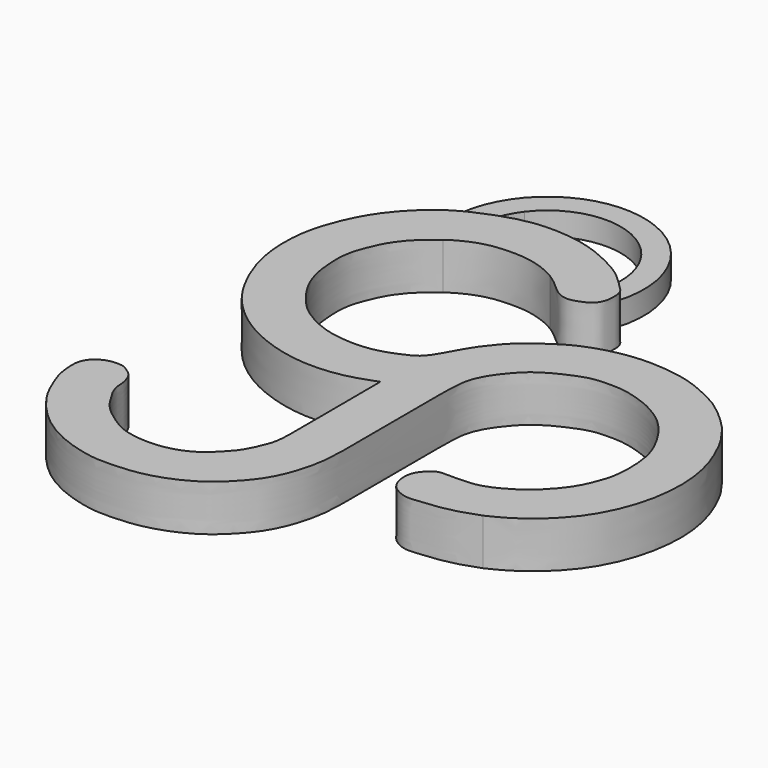
from build123d import *

# Parameters (mm, degrees)
F1_DEPTH = 6
F2_DEPTH = 3


with BuildPart() as f1:
    # F0 (on Top) → F1 (new body)
    with BuildSketch(Plane.XY):
        with BuildLine():
            add(Edge.make_bspline(
                [(-61.713565141, -18.9343132079), (-63.0146348838, -19.4095390469), (-65.733189771, -20.4025123556), (-70.8280130497, -20.6815591765), (-75.7018481976, -19.5041294338), (-80.0931153376, -17.3641610679), (-84.0038443733, -13.8752753533), (-86.4313989815, -9.8518831116), (-88.2796036438, -5.0190108695), (-88.4963736266, 0.0085689786), (-87.8617186152, 3.6375292768), (-86.1935172065, 7.9287613179), (-83.9416658783, 11.1542399806), (-82.1275636618, 12.9283614758), (-81.3241270743, 13.5947379823)],
                knots=[0, 0, 0, 0, 0.0181122524, 0.0378370444, 0.0574807634, 0.0768858202, 0.0968162077, 0.1158466157, 0.1358456208, 0.1553780521, 0.1722749914, 0.190949199, 0.2090855796, 0.2233461087, 0.2233461087, 0.2233461087, 0.2233461087], degree=3))
            add(Edge.make_bspline(
                [(-35.296164453, -35.3126786649), (-35.8181301783, -35.5024037361), (-36.8134666802, -35.8641904962), (-38.0708117456, -36.270480159), (-40.138121174, -36.7077930279), (-42.3688721513, -36.8892351142), (-44.2325900627, -37.1059998289), (-45.7225874453, -36.2585038344), (-46.2929253284, -35.686129434), (-46.7363136163, -34.8014748443), (-46.8692619716, -33.8262575164), (-46.8065307463, -32.7032975926), (-46.2297636494, -31.7451552895), (-45.5431628055, -31.0933682437), (-44.8464319505, -30.5974831217), (-43.7455158564, -30.5822460272), (-42.5044985041, -30.6260654275), (-40.8703078904, -30.5481728825), (-39.8792195184, -30.4326386682), (-38.1797456225, -29.8531864623), (-36.9342661804, -29.1089567426), (-35.3238356448, -28.1904757097), (-33.170383713, -26.07435277), (-31.8582431136, -24.2273615637), (-31.1469842445, -22.6450405096), (-30.3725491148, -20.5779895244), (-30.2104838527, -18.4841397494), (-30.2501485523, -16.3106662094), (-30.6343803225, -13.9306564773), (-31.7748028839, -11.5465745257), (-33.186348835, -9.4322593089), (-34.8104844807, -7.735799033), (-37.1662119159, -6.2493083282), (-39.2182087251, -5.5030771293), (-41.166575858, -4.9558334521), (-42.9870195119, -4.859445306), (-45.4834836068, -4.897725137), (-47.7441223228, -5.8310077864), (-49.5208260418, -6.6596538791), (-51.4234507273, -7.8666605714), (-53.073082843, -9.7195908219), (-54.248737469, -11.3737650388), (-54.997105148, -13.1154447546), (-55.2687748261, -15.0229815759), (-55.2632841388, -20.2243601486), (-55.2042759513, -27.8226519462), (-55.2098481, -33.936082992), (-55.4095257107, -36.7774227554), (-56.4540380047, -40.5834941392), (-57.9776164972, -43.2587210437), (-59.7304487982, -45.2135126916), (-61.4142605805, -46.8277136166), (-63.9910912681, -48.4006874678), (-66.4861437494, -49.3100674413), (-68.5320453717, -49.8112197331), (-70.8281422598, -50.0305338543), (-73.6749221598, -50.1055434421), (-76.0600796044, -49.5953323554), (-78.2545980933, -48.9285309184), (-80.3394186289, -47.94916046), (-82.3766699977, -46.6394319711), (-84.5941350037, -44.5319080526), (-86.5559834995, -41.9402439855), (-87.7388820002, -38.9490920475), (-88.223461995, -37.5450863847), (-88.4518870314, -35.3054185599), (-88.1689144899, -33.996902953), (-87.2535647901, -32.9598891209), (-86.064578952, -32.4525417401), (-85.2012031694, -32.3805571825), (-84.1562979368, -32.3779337124), (-83.4415258264, -32.8900691989), (-82.5667565857, -33.4633434329), (-82.1276496152, -34.4287627257), (-81.8786209528, -35.3072880017), (-81.9010780662, -36.2685272173), (-81.5687414202, -37.3678700953), (-80.9293520817, -38.5113387996), (-79.7039044506, -40.4301147847), (-78.1143566296, -41.6772916231), (-75.8736928043, -43.2904010822), (-73.2240783852, -43.8825156923), (-70.3458122862, -43.9330397612), (-67.705309963, -43.1744317274), (-65.9148021977, -42.0895899621), (-64.485842596, -40.641590991), (-63.208787924, -39.2372686238), (-62.2393015406, -37.055484543), (-61.6280736511, -35.274776599), (-61.6970903399, -31.4658620455), (-61.6611319259, -25.6158249209), (-61.6957177272, -21.2085911438), (-61.713565141, -18.9343132079)],
                knots=[0, 0, 0, 0, 0.009713792, 0.018523231, 0.0296177616, 0.0412426231, 0.0517266457, 0.0614301399, 0.0683058968, 0.0757330625, 0.0833730649, 0.0914304993, 0.0994611402, 0.1069060689, 0.1138295582, 0.1216652726, 0.1304187819, 0.1401051374, 0.1479141307, 0.1580048595, 0.167282029, 0.177666793, 0.1910473747, 0.2026102156, 0.2126450904, 0.2239459464, 0.2350754304, 0.2463460933, 0.25821468, 0.2706831301, 0.2828675446, 0.2946370949, 0.3073617348, 0.3187773159, 0.3295233224, 0.3398791347, 0.351949174, 0.3639146961, 0.3746414794, 0.3860925584, 0.3981828339, 0.4091672758, 0.4194298037, 0.4298025383, 0.4470568677, 0.4688647684, 0.4876514078, 0.5005796386, 0.5155842151, 0.5291606332, 0.5414036299, 0.5531147539, 0.5664213601, 0.5789541197, 0.5899760135, 0.6016125951, 0.6145640928, 0.6265689317, 0.6381339955, 0.6497018232, 0.6616027915, 0.6749535609, 0.6890266756, 0.7025518969, 0.7120828724, 0.7233651725, 0.7322075404, 0.7410057732, 0.7495979039, 0.7567898106, 0.7644154198, 0.7715498147, 0.7793119137, 0.7871135756, 0.7944144135, 0.8018723941, 0.8099307547, 0.8187750089, 0.8302047394, 0.8412351794, 0.8538198609, 0.8664300361, 0.8794483478, 0.8920813992, 0.9031266466, 0.9139306713, 0.9245683387, 0.9362211561, 0.9466401074, 0.9612753029, 0.9800167795, 1, 1, 1, 1], degree=3))
            add(Edge.make_bspline(
                [(-27.7324169874, -6.1554475687), (-27.5844867603, -6.3458762594), (-27.2377225254, -6.792261427), (-26.4338168242, -8.0377056958), (-26.1060869313, -8.7749670887), (-25.5946712876, -9.7786394426), (-25.0191857066, -11.1493826388), (-24.4811088291, -12.7162052178), (-24.1042796832, -14.4700558507), (-23.8285203007, -16.4444047718), (-23.8374285511, -18.7169653805), (-24.1293597245, -21.3072211445), (-24.7941702457, -23.9050809113), (-25.8118469154, -26.437426106), (-27.3504709137, -29.134360782), (-29.8206777102, -31.8218017139), (-32.2980131944, -33.794270527), (-34.2746658689, -34.8260445424), (-35.296164453, -35.3126786649)],
                knots=[0, 0, 0, 0, 0.0390972492, 0.0916538163, 0.1313091765, 0.1765217524, 0.2298017258, 0.2858828672, 0.3440053241, 0.405212187, 0.4707281208, 0.5409912037, 0.6121141795, 0.6835800727, 0.7602162872, 0.8430639552, 0.9205274895, 1, 1, 1, 1], degree=3))
            add(Edge.make_bspline(
                [(-76.2045055318, 9.3074033652), (-76.5218089854, 9.078997831), (-77.3773037078, 8.4142063955), (-78.6357294598, 7.2936101698), (-80.0849730461, 5.4657053706), (-81.0194176934, 3.4597682952), (-81.7898287642, 1.4029441494), (-82.0027625241, -0.6427525487), (-81.8251370277, -2.7335750938), (-81.6554744679, -4.303900693), (-80.9754892278, -6.350547843), (-80.0698438514, -7.9318516488), (-78.9522131255, -9.5079907124), (-77.6731560568, -10.9366966539), (-76.0414056738, -12.1577177333), (-74.0597869131, -13.1512858627), (-72.1184957982, -13.7994659129), (-69.7967649674, -14.0708597413), (-67.6883106362, -14.0507143955), (-65.5177403296, -13.6306348883), (-63.3791081133, -12.7167926114), (-61.9793247667, -12.0131728726), (-60.7552359052, -10.2374244527), (-59.2871040846, -7.2665300949), (-56.9416232761, -4.307658848), (-54.696689077, -2.5388777859), (-51.9338279159, -0.5945232282), (-48.7844052072, 0.6408205746), (-45.6888475134, 1.2953502861), (-42.9200856358, 1.4551420776), (-40.1957117703, 1.2302845705), (-38.1625579987, 0.849082493), (-36.7550362077, 0.3994965104), (-34.9638669841, -0.3245907992), (-32.9461903075, -1.3185776658), (-31.3698386362, -2.4415469665), (-29.7192270514, -3.8628099901), (-28.5410352847, -5.0717218964), (-27.9709637085, -5.8049874455), (-27.7324169874, -6.1554475687)],
                knots=[0.5206714775, 0.5206714775, 0.5206714775, 0.5206714775, 0.5277336201, 0.5401564435, 0.5535019976, 0.5666432084, 0.5796081177, 0.5922587254, 0.6048786406, 0.6160176421, 0.6287808902, 0.640757391, 0.6529111024, 0.6650704989, 0.6776165481, 0.6906636666, 0.7032847174, 0.7166603162, 0.7294334063, 0.7425600138, 0.7559227599, 0.7667307379, 0.7792767658, 0.7954759623, 0.812542903, 0.8274370589, 0.8434835205, 0.8597213359, 0.8753164124, 0.8900000858, 0.9045816478, 0.9171308213, 0.9277184173, 0.939911376, 0.953119681, 0.9654510177, 0.9784179337, 0.9898905772, 1, 1, 1, 1], degree=3))
            add(Edge.make_bspline(
                [(-77.7812605681, 15.8198985313), (-77.7656474583, 15.6184901087), (-77.6996325647, 14.8752566882), (-77.5241918195, 13.6648439941), (-77.1656405971, 12.1481399625), (-76.7845693515, 10.7825369702), (-76.4108544823, 9.7727883648), (-76.2045055318, 9.3074033652)],
                knots=[0.2819929467, 0.2819929467, 0.2819929467, 0.2819929467, 0.2893287156, 0.308895452, 0.3282423501, 0.3474354454, 0.3648385459, 0.3648385459, 0.3648385459, 0.3648385459], degree=3))
            add(Edge.make_bspline(
                [(-78.7460588266, 15.3344307924), (-78.4590934981, 15.48874223), (-78.1404400268, 15.6492648888), (-77.8021928593, 15.8099870355), (-77.781260567, 15.8198985311)],
                knots=[0.2382511161, 0.2382511161, 0.2382511161, 0.2382511161, 0.2428638243, 0.2431669836, 0.2431669836, 0.2431669836, 0.2431669836], degree=3))
            add(Edge.make_bspline(
                [(-81.3241270743, 13.5947379823), (-81.1414694644, 13.7462356136), (-80.3005582565, 14.4155061862), (-79.4716325774, 14.9442640461), (-78.7460588266, 15.3344307924)],
                knots=[0.2233461087, 0.2233461087, 0.2233461087, 0.2233461087, 0.2265881743, 0.2382511161, 0.2382511161, 0.2382511161, 0.2382511161], degree=3))
        make_face()
        with BuildLine():
            add(Edge.make_bspline(
                [(-77.781260567, 15.8198985311), (-76.4931380597, 16.4298279359), (-73.4700030416, 17.6078829506), (-69.6860075919, 18.1664098839), (-65.2210105766, 17.8453428936), (-62.7141483006, 16.958191199), (-61.4468064845, 16.3875784567)],
                knots=[0.2431669836, 0.2431669836, 0.2431669836, 0.2431669836, 0.2618226723, 0.2792369205, 0.2976021198, 0.3152672972, 0.3152672972, 0.3152672972, 0.3152672972], degree=3))
            add(Edge.make_bspline(
                [(-77.7812605681, 15.8198985313), (-77.7656474583, 15.6184901087), (-77.6996325647, 14.8752566882), (-77.5241918195, 13.6648439941), (-77.1656405971, 12.1481399625), (-76.7845693515, 10.7825369702), (-76.4108544823, 9.7727883648), (-76.2045055318, 9.3074033652)],
                knots=[0.2819929467, 0.2819929467, 0.2819929467, 0.2819929467, 0.2893287156, 0.308895452, 0.3282423501, 0.3474354454, 0.3648385459, 0.3648385459, 0.3648385459, 0.3648385459], degree=3))
            add(Edge.make_bspline(
                [(-62.8149353652, 9.903892193), (-63.1530114927, 10.112592561), (-64.2933964119, 10.7297810382), (-66.3964523357, 11.3795145378), (-68.6035228421, 11.5841795565), (-71.455591251, 11.471487449), (-73.6670237686, 10.7636861036), (-75.1235336284, 10.0489853203), (-75.9487774766, 9.4914848884), (-76.2045055318, 9.3074033652)],
                knots=[0.4405103361, 0.4405103361, 0.4405103361, 0.4405103361, 0.4469402161, 0.4612733738, 0.4744485529, 0.4892298533, 0.5026357823, 0.5149798029, 0.5206714775, 0.5206714775, 0.5206714775, 0.5206714775], degree=3))
            add(Edge.make_bspline(
                [(-62.8149353652, 9.903892193), (-62.7099626128, 10.1750316236), (-62.4315811932, 10.9625624816), (-62.1007460311, 12.1481399625), (-61.7421948087, 13.6648439941), (-61.5402877605, 15.0578548019), (-61.4689217957, 16.0066300277), (-61.4468064841, 16.3875784568)],
                knots=[0.6191083522, 0.6191083522, 0.6191083522, 0.6191083522, 0.6291365538, 0.6483296491, 0.6676765471, 0.6872432836, 0.7015560561, 0.7015560561, 0.7015560561, 0.7015560561], degree=3))
        make_face()
        with BuildLine():
            add(Edge.make_bspline(
                [(-61.4468064845, 16.3875784567), (-61.4387210484, 16.3839380396), (-61.0825686276, 16.22337035), (-60.7233153737, 16.0521064438), (-60.377706703, 15.8772837247)],
                knots=[0.3152672972, 0.3152672972, 0.3152672972, 0.3152672972, 0.3153799981, 0.3202306654, 0.3202306654, 0.3202306654, 0.3202306654], degree=3))
            add(Edge.make_bspline(
                [(-62.8149353652, 9.903892193), (-62.7099626128, 10.1750316236), (-62.4315811932, 10.9625624816), (-62.1007460311, 12.1481399625), (-61.7421948087, 13.6648439941), (-61.5402877605, 15.0578548019), (-61.4689217957, 16.0066300277), (-61.4468064841, 16.3875784568)],
                knots=[0.6191083522, 0.6191083522, 0.6191083522, 0.6191083522, 0.6291365538, 0.6483296491, 0.6676765471, 0.6872432836, 0.7015560561, 0.7015560561, 0.7015560561, 0.7015560561], degree=3))
            add(Edge.make_bspline(
                [(-57.7184766628, 14.2386218759), (-57.1040316706, 13.7484886091), (-56.2385922947, 12.8208118517), (-54.9882083885, 11.7392577457), (-54.8634453308, 10.4745706289), (-54.9598637888, 9.0402785981), (-55.6680644185, 7.9861319672), (-56.710582305, 7.454319038), (-58.3291660915, 6.8691938499), (-60.0035771408, 7.5037817098), (-61.3488520287, 8.8906439946), (-62.4017038079, 9.6487970501), (-62.8149353652, 9.903892193)],
                knots=[0.3342753119, 0.3342753119, 0.3342753119, 0.3342753119, 0.3464829764, 0.3575391041, 0.367165013, 0.3776473327, 0.3872383492, 0.3967041143, 0.4079608764, 0.4193316329, 0.4326510727, 0.4405103361, 0.4405103361, 0.4405103361, 0.4405103361], degree=3))
            add(Edge.make_bspline(
                [(-60.377706703, 15.8772837247), (-59.4621787455, 15.4141729859), (-58.5035884124, 14.8508669845), (-57.7786283134, 14.2866039172), (-57.7184766628, 14.2386218759)],
                knots=[0.3202306654, 0.3202306654, 0.3202306654, 0.3202306654, 0.3330802314, 0.3342753119, 0.3342753119, 0.3342753119, 0.3342753119], degree=3))
        make_face()
    extrude(amount=F1_DEPTH)

    # F0 (on Top) → F2 (join)
    with BuildSketch(Plane.XY):
        with BuildLine():
            ThreePointArc((-57.7184766628, 14.2386218759), (-58.3193846113, 23.3336305696), (-64.9360002166, 29.6026553289))
            add(Edge.make_bspline(
                [(-62.0849376344, 23.7871187501), (-62.0925733957, 23.817134584), (-62.2244672864, 24.3327717422), (-62.5063607695, 25.3429873926), (-63.1472614927, 27.0385998339), (-64.014977683, 28.5182448026), (-64.6487121355, 29.2864815447), (-64.9336220661, 29.6000403925), (-64.9360002166, 29.6026553289)],
                knots=[0.798733913, 0.798733913, 0.798733913, 0.798733913, 0.799917792, 0.8191108873, 0.8401182393, 0.860681824, 0.8790023039, 0.8791565789, 0.8791565789, 0.8791565789, 0.8791565789], degree=3))
            ThreePointArc((-62.0849376343, 23.7871187501), (-60.3470309595, 20.0230635373), (-60.377706703, 15.8772837247))
            add(Edge.make_bspline(
                [(-60.377706703, 15.8772837247), (-59.4621787455, 15.4141729859), (-58.5035884124, 14.8508669845), (-57.7786283134, 14.2866039172), (-57.7184766628, 14.2386218759)],
                knots=[0.3202306654, 0.3202306654, 0.3202306654, 0.3202306654, 0.3330802314, 0.3342753119, 0.3342753119, 0.3342753119, 0.3342753119], degree=3))
        make_face()
        with BuildLine():
            ThreePointArc((-64.9360002166, 29.6026553289), (-69.6331933141, 30.518770963), (-74.3303864116, 29.6026553289))
            add(Edge.make_bspline(
                [(-74.3303864116, 29.6026553289), (-74.3327645621, 29.6000403925), (-74.6176744927, 29.2864815447), (-75.2514089452, 28.5182448026), (-76.1191251354, 27.0385998339), (-76.7600258586, 25.3429873926), (-77.0419193418, 24.3327717422), (-77.1738132324, 23.817134584), (-77.1814489938, 23.7871187501)],
                knots=[0.0974154203, 0.0974154203, 0.0974154203, 0.0974154203, 0.0975696953, 0.1158901752, 0.1364537599, 0.1574611118, 0.1766542072, 0.1778380862, 0.1778380862, 0.1778380862, 0.1778380862], degree=3))
            ThreePointArc((-77.1814489938, 23.7871187501), (-69.6331933141, 27.518770963), (-62.0849376343, 23.7871187501))
            add(Edge.make_bspline(
                [(-62.0849376344, 23.7871187501), (-62.0925733957, 23.817134584), (-62.2244672864, 24.3327717422), (-62.5063607695, 25.3429873926), (-63.1472614927, 27.0385998339), (-64.014977683, 28.5182448026), (-64.6487121355, 29.2864815447), (-64.9336220661, 29.6000403925), (-64.9360002166, 29.6026553289)],
                knots=[0.798733913, 0.798733913, 0.798733913, 0.798733913, 0.799917792, 0.8191108873, 0.8401182393, 0.860681824, 0.8790023039, 0.8791565789, 0.8791565789, 0.8791565789, 0.8791565789], degree=3))
        make_face()
        with BuildLine():
            ThreePointArc((-74.3303864116, 29.6026553289), (-81.0877133791, 23.0231660392), (-81.3241270743, 13.5947379823))
            add(Edge.make_bspline(
                [(-81.3241270743, 13.5947379823), (-81.1414694644, 13.7462356136), (-80.3005582565, 14.4155061862), (-79.4716325774, 14.9442640461), (-78.7460588266, 15.3344307924)],
                knots=[0.2233461087, 0.2233461087, 0.2233461087, 0.2233461087, 0.2265881743, 0.2382511161, 0.2382511161, 0.2382511161, 0.2382511161], degree=3))
            ThreePointArc((-78.7460588266, 15.3344307924), (-78.9745113834, 19.7478680473), (-77.1814489938, 23.7871187501))
            add(Edge.make_bspline(
                [(-74.3303864116, 29.6026553289), (-74.3327645621, 29.6000403925), (-74.6176744927, 29.2864815447), (-75.2514089452, 28.5182448026), (-76.1191251354, 27.0385998339), (-76.7600258586, 25.3429873926), (-77.0419193418, 24.3327717422), (-77.1738132324, 23.817134584), (-77.1814489938, 23.7871187501)],
                knots=[0.0974154203, 0.0974154203, 0.0974154203, 0.0974154203, 0.0975696953, 0.1158901752, 0.1364537599, 0.1574611118, 0.1766542072, 0.1778380862, 0.1778380862, 0.1778380862, 0.1778380862], degree=3))
        make_face()
    extrude(amount=F2_DEPTH)


solid = f1.part
